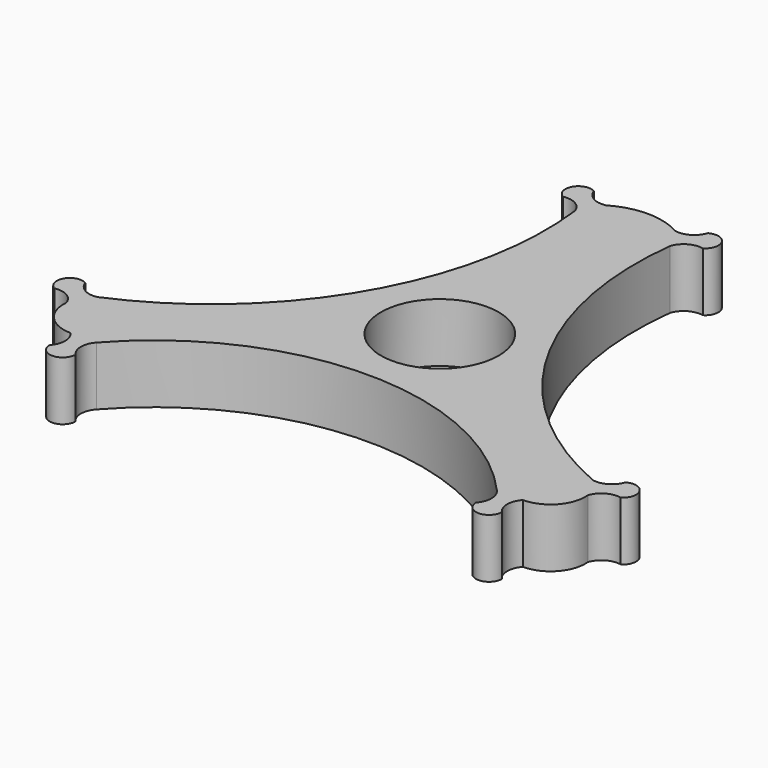
from build123d import *

# Parameters (mm, degrees)
F0_R     = 15
F0_R_2   = 10
F1_DEPTH = 10


# Not quite as in the source:
# - a feature names something its author has since deleted; it is built from what else it names


with BuildPart() as f1:
    # F0 (on Top) → F1 (new body)
    with BuildSketch(Plane.XY):
        with BuildLine():
            ThreePointArc((42.0721931458, -20.106328072), (15.2726376348, 3.6807596445), (8.0721931458, 38.7833993854))
            ThreePointArc((8.0721931458, 38.7833993854), (9.5591074328, 40.6079882936), (11.8827049224, 40.9833993854))
            ThreePointArc((11.8827049224, 40.9833993854), (12.6879608107, 43.9886552737), (9.6827049224, 44.793911162))
            ThreePointArc((9.6827049224, 44.793911162), (8.1957906353, 42.9693222537), (5.8721931458, 42.593911162))
            ThreePointArc((5.8721931458, 42.593911162), (0, 44.17956576), (-5.8721931458, 42.593911162))
            ThreePointArc((-5.8721931458, 42.593911162), (-8.1957906353, 42.9693222537), (-9.6827049224, 44.793911162))
            ThreePointArc((-9.6827049224, 44.793911162), (-12.6879608107, 43.9886552737), (-11.8827049224, 40.9833993854))
            ThreePointArc((-11.8827049224, 40.9833993854), (-9.5591074328, 40.6079882936), (-8.0721931458, 38.7833993854))
            ThreePointArc((-8.0721931458, 38.7833993854), (-15.2726376348, 3.6807596445), (-42.0721931458, -20.106328072))
            ThreePointArc((-42.0721931458, -20.106328072), (-44.3957906353, -19.7309169803), (-45.8827049224, -17.906328072))
            ThreePointArc((-45.8827049224, -17.906328072), (-48.8879608107, -18.7115839603), (-48.0827049224, -21.7168398486))
            ThreePointArc((-48.0827049224, -21.7168398486), (-45.7591074328, -22.0922509404), (-44.2721931458, -23.9168398486))
            ThreePointArc((-44.2721931458, -23.9168398486), (-42.7651143596, -28.4458898793), (-38.4, -30.3770442686))
            ThreePointArc((-38.4, -30.3770442686), (-37.5391516656, -32.6039224965), (-38.4, -34.8308007245))
            ThreePointArc((-38.4, -34.8308007245), (-36.2, -37.010864664), (-34, -34.8308007245))
            ThreePointArc((-34, -34.8308007245), (-34.8608483344, -32.6039224965), (-34, -30.3770442686))
            ThreePointArc((-34, -30.3770442686), (0, -15.1188267986), (34, -30.3770442686))
            ThreePointArc((34, -30.3770442686), (34.8608483344, -32.6039224965), (34, -34.8308007245))
            ThreePointArc((34, -34.8308007245), (36.2, -37.010864664), (38.4, -34.8308007245))
            ThreePointArc((38.4, -34.8308007245), (37.5391516656, -32.6039224965), (38.4, -30.3770442686))
            ThreePointArc((38.4, -30.3770442686), (42.7651143596, -28.4458898793), (44.2721931458, -23.9168398486))
            ThreePointArc((44.2721931458, -23.9168398486), (45.7591074328, -22.0922509404), (48.0827049224, -21.7168398486))
            ThreePointArc((48.0827049224, -21.7168398486), (48.8879608107, -18.7115839603), (45.8827049224, -17.906328072))
            ThreePointArc((45.8827049224, -17.906328072), (44.3957906353, -19.7309169803), (42.0721931458, -20.106328072))
        make_face()
        Circle(F0_R, mode=Mode.SUBTRACT)
        Circle(F0_R)
        Circle(F0_R_2, mode=Mode.SUBTRACT)
    extrude(amount=F1_DEPTH)


solid = f1.part
